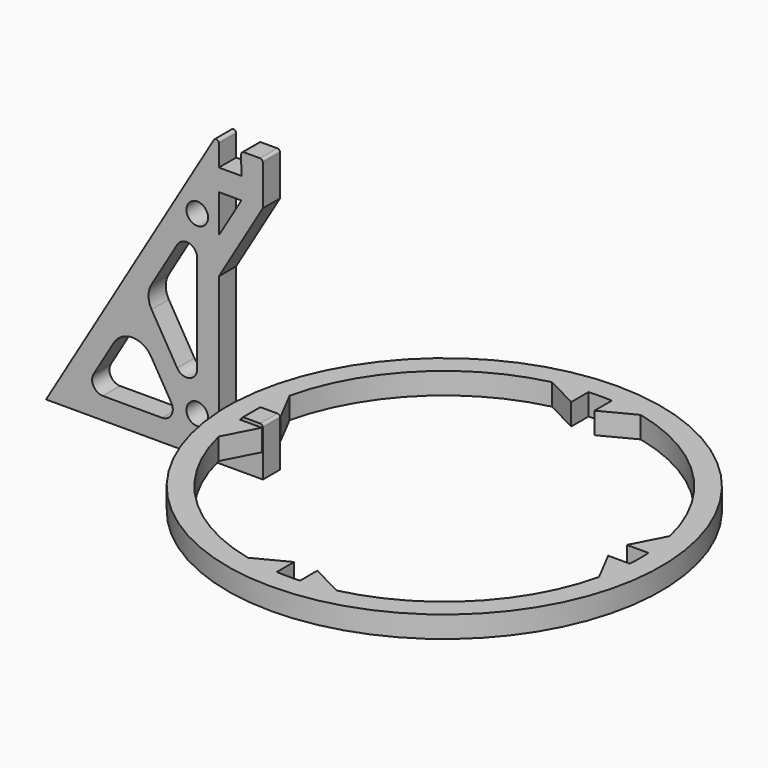
from build123d import *

# Parameters (mm, degrees)
F0_R            = 3.175
F1_DEPTH        = 3.175
F3_DEPTH        = 6.35
F6_DEPTH        = 6.35
F6_COPIES_COUNT = 4


# Not quite as in the source:
# - a pattern or mirror of a feature is missing from the dataset's text; its kind, count and spacing are read off the source's solid


with BuildPart() as f1:
    # F0 (on Front) → F1 (new body, symmetric)
    with BuildSketch(Plane.XZ):
        with BuildLine():
            Line((-114.554, 0), (-63.754, 0))
            Line((-63.754, 0), (-57.15, 0))
            Line((-57.15, 0), (-50.8, 0))
            Line((-50.8, 0), (-50.8, 7.1307474974))
            Line((-50.8, 7.1307474974), (-50.8, 13.4807474974))
            ThreePointArc((-50.8, 13.4807474974), (-51.0286756476, 14.0328193472), (-51.5807474974, 14.2614949948))
            Line((-51.5807474974, 14.2614949948), (-56.3692525026, 14.2614949948))
            ThreePointArc((-56.3692525026, 14.2614949948), (-56.9213243524, 14.0328193472), (-57.15, 13.4807474974))
            Line((-57.15, 13.4807474974), (-57.15, 7.1307474974))
            Line((-57.15, 7.1307474974), (-63.754, 7.1307474974))
            Line((-63.754, 7.1307474974), (-63.754, 48.4004353356))
            Line((-63.754, 48.4004353356), (-50.832637261, 70.2052349577))
            Line((-50.832637261, 70.2052349577), (-50.832637261, 82.1244455233))
            ThreePointArc((-50.832637261, 82.1244455233), (-51.0613129086, 82.6765173731), (-51.6133847584, 82.9051930207))
            Line((-51.6133847584, 82.9051930207), (-56.3978665697, 82.9051930207))
            ThreePointArc((-56.3978665697, 82.9051930207), (-56.9513553502, 82.6750967964), (-57.1786037546, 82.120432695))
            Line((-57.1786037546, 82.120432695), (-57.15, 76.5552768946))
            Line((-57.15, 76.5552768946), (-63.754, 76.5552768946))
            Line((-63.754, 76.5552768946), (-63.754, 82.8760177533))
            ThreePointArc((-63.754, 82.8760177533), (-64.3283963131, 83.629002377), (-65.2064179593, 83.2740446937))
            Line((-65.2064179593, 83.2740446937), (-114.554, 0))
        make_face()
        with BuildLine():
            ThreePointArc((-97.837727428, 6.35), (-100.5963277724, 7.9531383205), (-100.5691530473, 11.1436225892))
            Line((-100.5691530473, 11.1436225892), (-94.6168512386, 21.1881318914))
            ThreePointArc((-94.6168512386, 21.1881318914), (-89.154, 24.300886713), (-83.6911487614, 21.1881318914))
            Line((-83.6911487614, 21.1881318914), (-77.7388469527, 11.1436225892))
            ThreePointArc((-77.7388469527, 11.1436225892), (-77.7116722276, 7.9531383205), (-80.470272572, 6.35))
            Line((-80.470272572, 6.35), (-97.837727428, 6.35))
        make_face(mode=Mode.SUBTRACT)
        with Locations((-70.104, 10.715625)):
            Circle(F0_R, mode=Mode.SUBTRACT)
        with BuildLine():
            ThreePointArc((-75.9631742143, 52.6662118698), (-72.4211622502, 54.0981405316), (-70.104, 51.0605382613))
            Line((-70.104, 51.0605382613), (-70.104, 22.3013408218))
            ThreePointArc((-70.104, 22.3013408218), (-72.4398490426, 19.2392417589), (-76.0104256193, 20.6827182325))
            Line((-76.0104256193, 20.6827182325), (-83.545023111, 33.3973514998))
            ThreePointArc((-83.545023111, 33.3973514998), (-84.4321718724, 36.6345966782), (-83.545023111, 39.8718418567))
            Line((-83.545023111, 39.8718418567), (-75.9631742143, 52.6662118698))
        make_face(mode=Mode.SUBTRACT)
        with Locations((-70.104, 62.5535683565)):
            Circle(F0_R, mode=Mode.SUBTRACT)
        Polygon((-63.754, 59.0059507892), (-63.754, 70.2052768946), (-57.1173623079, 70.2052768946), align=None, mode=Mode.SUBTRACT)
    extrude(amount=F1_DEPTH, both=True)


with BuildPart() as f3:
    # F2 (on face) → F3 (new body)
    with BuildSketch(Plane.XY.offset(7.1307474974)):
        with BuildLine():
            ThreePointArc((-63.6748921554, -3.175), (1.5879926835, -63.7342199704), (63.754, 0))
            ThreePointArc((63.754, 0), (1.5879926835, 63.7342199704), (-63.6748921554, 3.175))
            Line((-63.6748921554, 3.175), (-57.3161288542, 3.175))
            ThreePointArc((-57.3161288542, 3.175), (1.5881078673, 57.3820282426), (57.4040003121, 0))
            ThreePointArc((57.4040003121, 0), (1.5881078673, -57.3820282426), (-57.3161288542, -3.175))
            Line((-57.3161288542, -3.175), (-63.6748921554, -3.175))
        make_face()
        with BuildLine():
            Line((-57.3161288542, 3.175), (-63.6748921554, 3.175))
            ThreePointArc((-63.6748921554, 3.175), (-63.7342199704, 1.5879926835), (-63.754, 0))
            ThreePointArc((-63.754, 0), (-63.7342199704, -1.5879926835), (-63.6748921554, -3.175))
            Line((-63.6748921554, -3.175), (-57.3161288542, -3.175))
            ThreePointArc((-57.3161288542, -3.175), (-57.4040003121, 0), (-57.3161288542, 3.175))
        make_face()
    extrude(amount=F3_DEPTH)

    # F5 (on face) → F6 (join, through all)
    with BuildSketch(Plane.XY.offset(13.4807474974)):
        with BuildLine():
            Line((-50.9316508603, -3.429), (-57.3014939668, -3.429))
            ThreePointArc((-57.3014939668, -3.429), (-56.806984466, -8.2574673909), (-55.9063426191, -13.0268993544))
            Line((-55.9063426191, -13.0268993544), (-50.9316508603, -3.429))
        make_face()
    f6 = extrude(amount=-F6_DEPTH)

    # F6_copies: F6 ×4 about axis
    f6_copies_axis = Axis((0, 0, 0), (0, 0, 1))
    for i in range(1, F6_COPIES_COUNT):
        add(f6.rotate(f6_copies_axis, i * 360 / F6_COPIES_COUNT))

    # F6_copies1: F6 across plane
    add(f6.mirror(Plane(origin=(0, 0, 0), x_dir=(0, 0, 1), z_dir=(1, 0, 0))))

    # F6_copies2: F6 across plane
    add(f6.mirror(Plane(origin=(0, 0, 0), x_dir=(-0.7071067812, -0.7071067812, 0), z_dir=(0.7071067812, -0.7071067812, 0))))

    # F6_copies3: F6 across plane
    add(f6.mirror(Plane(origin=(0, 0, 0), x_dir=(0.7071067812, -0.7071067812, 0), z_dir=(0.7071067812, 0.7071067812, 0))))

    # F6_copies4: F6 across plane
    add(f6.mirror(Plane.ZX))


solid = Compound([f1.part, f3.part])
